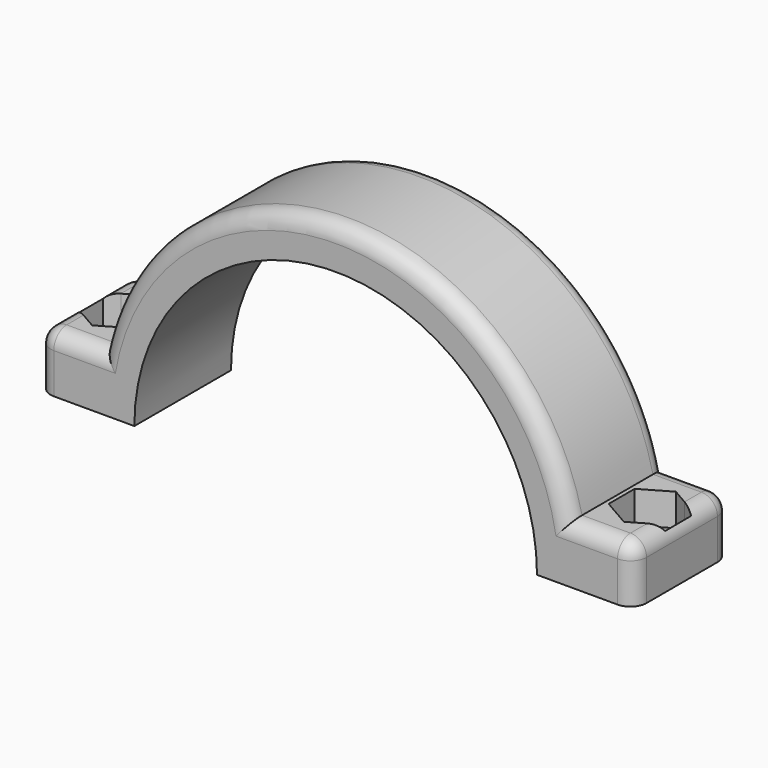
from build123d import *

# Parameters (mm, degrees)
F1_DEPTH  = 15
F2_R      = 2
F4_DEPTH  = 25
F5_DEPTH  = 4
F6_DEPTH  = 25
F8_DEPTH  = 25
F9_DEPTH  = 4
F10_DEPTH = 25


with BuildPart() as f1:
    # F0 (on Front) → F1 (new body)
    with BuildSketch(Plane.XZ):
        with BuildLine():
            ThreePointArc((-23.1304047869, 0.0265709655), (1.8676618749, 25.0246376273), (26.8657285366, 0.0265709655))
            Line((26.8657285366, 0.0265709655), (38.8657285366, 0.0265709655))
            Line((38.8657285366, 0.0265709655), (38.8657285366, 7.0265709655))
            Line((38.8657285366, 7.0265709655), (30.8657285366, 7.0265709655))
            ThreePointArc((30.8657285366, 7.0265709655), (1.8676618749, 30.1297350471), (-27.1304047869, 7.0265709655))
            Line((-27.1304047869, 7.0265709655), (-35.1304047869, 7.0265709655))
            Line((-35.1304047869, 7.0265709655), (-35.1304047869, 0.0265709655))
            Line((-35.1304047869, 0.0265709655), (-23.1304047869, 0.0265709655))
        make_face()
    extrude(amount=F1_DEPTH)

    # F2
    f2_edges = [f1.edges().sort_by_distance(p)[0] for p in [
        (1.867662, -15, 30.129735),
        (34.865729, -15, 7.026571),
        (38.865729, -15, 3.526571),
        (38.865729, -7.5, 7.026571),
        (-31.130405, -15, 7.026571),
        (-35.130405, -15, 3.526571),
        (-35.130405, -7.5, 7.026571),
        (1.867662, 0, 30.129735),
        (-31.130405, 0, 7.026571),
        (-35.130405, 0, 3.526571),
        (34.865729, 0, 7.026571),
        (38.865729, 0, 3.526571),
    ]]
    fillet(f2_edges, radius=F2_R)

    # F3 (on face) → F4 (cut)
    with BuildSketch(Plane.XY.offset(7.0265709655)):
        with BuildLine():
            ThreePointArc((36.8657285366, -7.7325071808), (36.875896312, -7.6164511554), (36.8792894082, -7.5))
            ThreePointArc((36.8792894082, -7.5), (36.875896312, -7.3835488446), (36.8657285366, -7.2674928192))
            Line((36.8657285366, -7.2674928192), (36.8657285366, -7.7325071808))
        make_face()
    extrude(amount=-F4_DEPTH, mode=Mode.SUBTRACT)

    # F3 (on face) → F5 (cut)
    with BuildSketch(Plane.XY.offset(7.0265709655)):
        with BuildLine():
            ThreePointArc((36.8657285366, -7.7325071808), (32.8792894082, -7.5), (36.8657285366, -7.2674928192))
            Line((36.8657285366, -7.2674928192), (36.8657285366, -4.6048032856))
            Line((36.8657285366, -4.6048032856), (34.8714804252, -3.45855566))
            Line((34.8714804252, -3.45855566), (31.3753914503, -5.4860406077))
            Line((31.3753914503, -5.4860406077), (31.3832004333, -9.5274849477))
            Line((31.3832004333, -9.5274849477), (34.8870983913, -11.54144434))
            Line((34.8870983913, -11.54144434), (36.8657285366, -10.3939784529))
            Line((36.8657285366, -10.3939784529), (36.8657285366, -7.7325071808))
        make_face()
        with BuildLine():
            ThreePointArc((36.8657285366, -7.2674928192), (36.875896312, -7.3835488446), (36.8792894082, -7.5))
            ThreePointArc((36.8792894082, -7.5), (36.875896312, -7.6164511554), (36.8657285366, -7.7325071808))
            Line((36.8657285366, -7.7325071808), (36.8657285366, -10.3939784529))
            Line((36.8657285366, -10.3939784529), (38.3831873661, -9.5139593923))
            Line((38.3831873661, -9.5139593923), (38.3753783831, -5.4725150523))
            Line((38.3753783831, -5.4725150523), (36.8657285366, -4.6048032856))
            Line((36.8657285366, -4.6048032856), (36.8657285366, -7.2674928192))
        make_face()
    extrude(amount=-F5_DEPTH, mode=Mode.SUBTRACT)

    # F3 (on face) → F6 (cut)
    with BuildSketch(Plane.XY.offset(7.0265709655)):
        with BuildLine():
            Line((36.8657285366, -7.7325071808), (36.8657285366, -7.2674928192))
            ThreePointArc((36.8657285366, -7.2674928192), (32.8792894082, -7.5), (36.8657285366, -7.7325071808))
        make_face()
    extrude(amount=-F6_DEPTH, mode=Mode.SUBTRACT)

    # F7 (on face) → F8 (cut)
    with BuildSketch(Plane.XY.offset(7.0265709655)):
        with BuildLine():
            ThreePointArc((-33.1304047869, -7.74764379), (-31.0207948898, -9.4935798639), (-29.1461082168, -7.4975095821))
            ThreePointArc((-29.1461082168, -7.4975095821), (-31.0207948898, -5.5014393002), (-33.1304047869, -7.2473753741))
            Line((-33.1304047869, -7.2473753741), (-33.1304047869, -7.74764379))
        make_face()
    extrude(amount=-F8_DEPTH, mode=Mode.SUBTRACT)

    # F7 (on face) → F9 (cut)
    with BuildSketch(Plane.XY.offset(7.0265709655)):
        with BuildLine():
            ThreePointArc((-33.1304047869, -7.74764379), (-33.1461082168, -7.4975095821), (-33.1304047869, -7.2473753741))
            Line((-33.1304047869, -7.2473753741), (-33.1304047869, -4.6022885965))
            Line((-33.1304047869, -4.6022885965), (-34.6500061748, -5.4835501898))
            Line((-34.6500061748, -5.4835501898), (-34.6421971917, -9.5249945298))
            Line((-34.6421971917, -9.5249945298), (-33.1304047869, -10.3939377894))
            Line((-33.1304047869, -10.3939377894), (-33.1304047869, -7.74764379))
        make_face()
        with BuildLine():
            ThreePointArc((-33.1304047869, -7.2473753741), (-31.0207948898, -5.5014393002), (-29.1461082168, -7.4975095821))
            ThreePointArc((-29.1461082168, -7.4975095821), (-31.0207948898, -9.4935798639), (-33.1304047869, -7.74764379))
            Line((-33.1304047869, -7.74764379), (-33.1304047869, -10.3939377894))
            Line((-33.1304047869, -10.3939377894), (-31.1382992338, -11.5389539221))
            Line((-31.1382992338, -11.5389539221), (-27.6422102589, -9.5114689744))
            Line((-27.6422102589, -9.5114689744), (-27.650019242, -5.4700246344))
            Line((-27.650019242, -5.4700246344), (-31.1539171999, -3.4560652421))
            Line((-31.1539171999, -3.4560652421), (-33.1304047869, -4.6022885965))
            Line((-33.1304047869, -4.6022885965), (-33.1304047869, -7.2473753741))
        make_face()
    extrude(amount=-F9_DEPTH, mode=Mode.SUBTRACT)

    # F7 (on face) → F10 (cut)
    with BuildSketch(Plane.XY.offset(7.0265709655)):
        with BuildLine():
            Line((-33.1304047869, -7.74764379), (-33.1304047869, -7.2473753741))
            ThreePointArc((-33.1304047869, -7.2473753741), (-33.1461082168, -7.4975095821), (-33.1304047869, -7.74764379))
        make_face()
    extrude(amount=-F10_DEPTH, mode=Mode.SUBTRACT)


solid = f1.part
